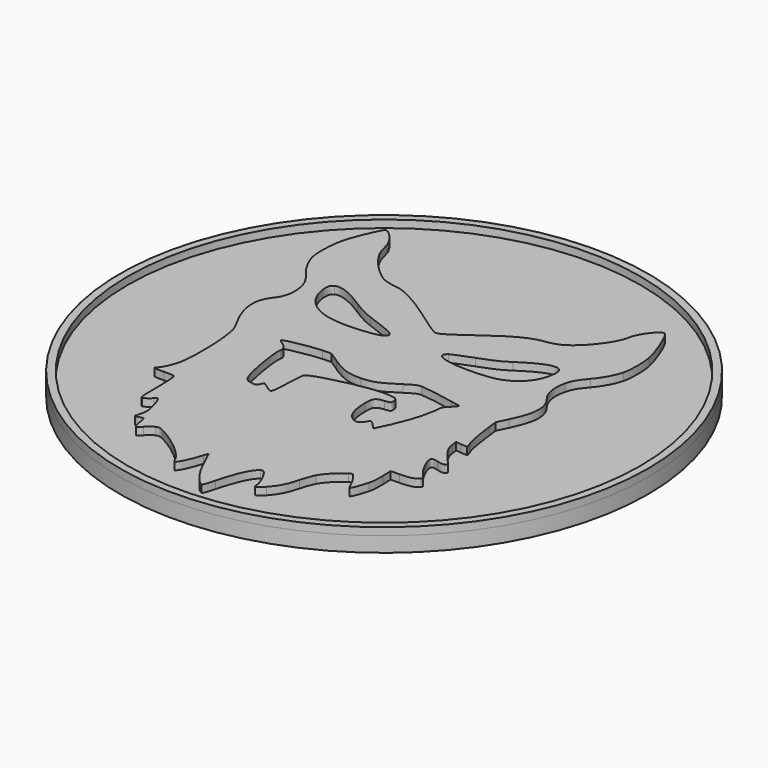
from build123d import *

# Parameters (mm, degrees)
F1_DEPTH = 1
F2_R     = 35
F3_DEPTH = 2
F4_R     = 35
F4_R_2   = 34
F5_DEPTH = 1


# Not quite as in the source:
# - ends of sketch curves that miss each other by under 0.0002 mm in the source are joined


with BuildPart() as f1:
    # F0 (on Top) → F1 (new body)
    with BuildSketch(Plane.XY):
        with BuildLine():
            Line((16.1826469271, 5.2708612479), (16.8400695237, 6.6341461731))
            add(Edge.make_bspline(
                [(16.9910679139, 12.732516303), (18.2577822603, 11.1594923939), (18.2164007999, 9.4882145174), (16.8400695237, 6.6341461731)],
                knots=[0, 0, 0, 0, 1, 1, 1, 1], degree=3))
            add(Edge.make_bspline(
                [(16.3616295009, 16.5726861761), (15.9908697191, 15.1813152196), (16.2392131876, 13.6661808871), (16.9910679139, 12.732516303)],
                knots=[0, 0, 0, 0, 1, 1, 1, 1], degree=3))
            add(Edge.make_bspline(
                [(17.7549925553, 18.9896539173), (16.8340840828, 17.8901305075), (16.608350267, 17.4985672419), (16.3616295009, 16.5726861761)],
                knots=[0, 0, 0, 0, 1, 1, 1, 1], degree=3))
            add(Edge.make_bspline(
                [(19.5483031014, 22.2723542054), (19.2596321814, 21.164071897), (18.6659092272, 20.0772477822), (17.7549925553, 18.9896539173)],
                knots=[0, 0, 0, 0, 1, 1, 1, 1], degree=3))
            add(Edge.make_bspline(
                [(19.5540287341, 26.4991346279), (19.8011714908, 25.3242562633), (19.7983403369, 23.2322956616), (19.5483031014, 22.2723542054)],
                knots=[0, 0, 0, 0, 1, 1, 1, 1], degree=3))
            add(Edge.make_bspline(
                [(17.3613460741, 31.7822766885), (17.7671351183, 31.7076772357), (19.1688004281, 28.330447016), (19.5540287341, 26.4991346279)],
                knots=[0, 0, 0, 0, 1, 1, 1, 1], degree=3))
            add(Edge.make_bspline(
                [(15.074723812, 28.6660865937), (15.2559545981, 29.8714277868), (16.741702099, 31.8961907452), (17.3613460741, 31.7822766885)],
                knots=[0, 0, 0, 0, 1, 1, 1, 1], degree=3))
            add(Edge.make_bspline(
                [(10.5930521191, 23.0509721747), (12.3876829908, 23.8999686358), (14.8154555549, 26.9417409854), (15.074723812, 28.6660865937)],
                knots=[0, 0, 0, 0, 1, 1, 1, 1], degree=3))
            add(Edge.make_bspline(
                [(8.8818992128, 22.5780426556), (9.427403017, 22.6472056597), (10.1781785803, 22.85470593), (10.5930521191, 23.0509721747)],
                knots=[0, 0, 0, 0, 1, 1, 1, 1], degree=3))
            add(Edge.make_bspline(
                [(1.7025667495, 18.7230730334), (5.4136975729, 21.4603613385), (7.0665795458, 22.3478826003), (8.8818992128, 22.5780426556)],
                knots=[0, 0, 0, 0, 1, 1, 1, 1], degree=3))
            add(Edge.make_bspline(
                [(-1.139369586, 17.0344307466), (-0.7369789819, 17.0344307466), (0.035244045, 17.4932769684), (1.7025667495, 18.7230730334)],
                knots=[0, 0, 0, 0, 1, 1, 1, 1], degree=3))
            add(Edge.make_bspline(
                [(-5.4533025812, 19.8115778984), (-2.3041017073, 17.5624688206), (-1.4838653366, 17.0344307466), (-1.139369586, 17.0344307466)],
                knots=[0, 0, 0, 0, 1, 1, 1, 1], degree=3))
            add(Edge.make_bspline(
                [(-8.5535875545, 21.720697149), (-7.7554292585, 21.3184456839), (-6.3603008446, 20.459341854), (-5.4533025812, 19.8115778984)],
                knots=[0, 0, 0, 0, 1, 1, 1, 1], degree=3))
            add(Edge.make_bspline(
                [(-11.0602009371, 22.5804912211), (-10.1866699201, 22.4741962137), (-9.7546933625, 22.3260237003), (-8.5535875545, 21.720697149)],
                knots=[0, 0, 0, 0, 1, 1, 1, 1], degree=3))
            add(Edge.make_bspline(
                [(-12.8320138873, 23.059260006), (-12.3873644201, 22.8418119108), (-11.7152713629, 22.6602027579), (-11.0602009371, 22.5804912211)],
                knots=[0, 0, 0, 0, 1, 1, 1, 1], degree=3))
            add(Edge.make_bspline(
                [(-16.2851561458, 26.3947741984), (-15.4734223835, 25.1582984045), (-13.7806207016, 23.5231600881), (-12.8320138873, 23.059260006)],
                knots=[0, 0, 0, 0, 1, 1, 1, 1], degree=3))
            add(Edge.make_bspline(
                [(-17.4473262444, 29.2439608911), (-17.0559172454, 27.7278100169), (-16.8846759732, 27.3079939642), (-16.2851561458, 26.3947741984)],
                knots=[0, 0, 0, 0, 1, 1, 1, 1], degree=3))
            add(Edge.make_bspline(
                [(-19.6386539259, 31.8102562987), (-19.0337263219, 31.8102562987), (-17.709473149, 30.2594038688), (-17.4473262444, 29.2439608911)],
                knots=[0, 0, 0, 0, 1, 1, 1, 1], degree=3))
            add(Edge.make_bspline(
                [(-21.5027325882, 27.6163899087), (-21.0601702065, 29.0864711639), (-19.8495088364, 31.8102562987), (-19.6386539259, 31.8102562987)],
                knots=[0, 0, 0, 0, 1, 1, 1, 1], degree=3))
            add(Edge.make_bspline(
                [(-21.74919724, 22.2310686119), (-22.0889620877, 23.4073232392), (-21.9668940617, 26.0745641014), (-21.5027325882, 27.6163899087)],
                knots=[0, 0, 0, 0, 1, 1, 1, 1], degree=3))
            add(Edge.make_bspline(
                [(-19.8346130445, 18.8263532445), (-20.7277127085, 19.8575266723), (-21.4183494276, 21.0856880736), (-21.74919724, 22.2310686119)],
                knots=[0, 0, 0, 0, 1, 1, 1, 1], degree=3))
            add(Edge.make_bspline(
                [(-18.7756283455, 17.195879164), (-18.9366280351, 17.6261934412), (-19.3608485153, 18.2793468794), (-19.8346130445, 18.8263532445)],
                knots=[0, 0, 0, 0, 1, 1, 1, 1], degree=3))
            add(Edge.make_bspline(
                [(-19.1345514591, 12.8525804454), (-18.3164443905, 13.9243594269), (-18.1780726475, 15.5987718895), (-18.7756283455, 17.195879164)],
                knots=[0, 0, 0, 0, 1, 1, 1, 1], degree=3))
            add(Edge.make_bspline(
                [(-20.0927388136, 10.3061527194), (-20.0912216529, 11.2790590836), (-19.8535934729, 11.9105845821), (-19.1345514591, 12.8525804454)],
                knots=[0, 0, 0, 0, 1, 1, 1, 1], degree=3))
            add(Edge.make_bspline(
                [(-18.5868828204, 5.7128167654), (-19.6253029115, 7.5160176163), (-20.0948470074, 8.9482768021), (-20.0927388136, 10.3061527194)],
                knots=[0, 0, 0, 0, 1, 1, 1, 1], degree=3))
            add(Edge.make_bspline(
                [(-17.7742137836, 3.1161301218), (-17.9802957504, 4.5409222382), (-18.0615731731, 4.8006232159), (-18.5868828204, 5.7128167654)],
                knots=[0, 0, 0, 0, 1, 1, 1, 1], degree=3))
            add(Edge.make_bspline(
                [(-17.7515684226, -4.5522716364), (-17.4512789538, -3.2317680053), (-17.4636851949, 0.9692171667), (-17.7742137836, 3.1161301218)],
                knots=[0, 0, 0, 0, 1, 1, 1, 1], degree=3))
            add(Edge.make_bspline(
                [(-18.8336035865, -6.9677459637), (-18.4850643607, -6.6784840106), (-17.9773312623, -5.5450502556), (-17.7515684226, -4.5522716364)],
                knots=[0, 0, 0, 0, 1, 1, 1, 1], degree=3))
            add(Edge.make_bspline(
                [(-17.7018741526, -7.3570784314), (-19.0362171041, -7.3929124486), (-19.2551487627, -7.3175965441), (-18.8336035865, -6.9677459637)],
                knots=[0, 0, 0, 0, 1, 1, 1, 1], degree=3))
            add(Edge.make_bspline(
                [(-16.2312680038, -7.6434167057), (-16.3592688758, -7.3277364549), (-16.3895737437, -7.3218366785), (-17.7018741526, -7.3570784314)],
                knots=[0, 0, 0, 0, 1, 1, 1, 1], degree=3))
            add(Edge.make_bspline(
                [(-16.0870003543, -10.6370017437), (-16.0944674236, -9.167807038), (-16.1593848404, -7.8206949583), (-16.2312680038, -7.6434167057)],
                knots=[0, 0, 0, 0, 1, 1, 1, 1], degree=3))
            add(Edge.make_bspline(
                [(-15.8719105864, -13.3085239015), (-16.0455582074, -13.3082600475), (-16.0753051119, -12.9388288587), (-16.0870003543, -10.6370017437)],
                knots=[0, 0, 0, 0, 1, 1, 1, 1], degree=3))
            add(Edge.make_bspline(
                [(-14.808504925, -12.599234109), (-15.0990701411, -12.9541719712), (-15.6308007644, -13.3088352493), (-15.8719105864, -13.3085239015)],
                knots=[0, 0, 0, 0, 1, 1, 1, 1], degree=3))
            add(Edge.make_bspline(
                [(-14.4542465749, -12.4327752793), (-14.5338604857, -12.3835703706), (-14.693277227, -12.4584773013), (-14.808504925, -12.599234109)],
                knots=[0, 0, 0, 0, 1, 1, 1, 1], degree=3))
            add(Edge.make_bspline(
                [(-13.6465008785, -14.7381748021), (-13.7897486442, -13.8486925771), (-14.2393005195, -12.5656191042), (-14.4542465749, -12.4327752793)],
                knots=[0, 0, 0, 0, 1, 1, 1, 1], degree=3))
            add(Edge.make_bspline(
                [(-13.8425972012, -16.7267398007), (-13.5642009335, -15.802671588), (-13.5303510987, -15.4594025828), (-13.6465008785, -14.7381748021)],
                knots=[0, 0, 0, 0, 1, 1, 1, 1], degree=3))
            add(Edge.make_bspline(
                [(-13.6206313971, -16.9565804166), (-13.9077388939, -17.0359609046), (-13.9290952399, -17.0138472975), (-13.8425972012, -16.7267398007)],
                knots=[0, 0, 0, 0, 1, 1, 1, 1], degree=3))
            add(Edge.make_bspline(
                [(-12.6213355831, -17.6683346059), (-12.7824700142, -16.6450057346), (-12.701721355, -16.702519407), (-13.6206313971, -16.9565804166)],
                knots=[0, 0, 0, 0, 1, 1, 1, 1], degree=3))
            add(Edge.make_bspline(
                [(-11.6474622818, -18.296259728), (-12.2924204136, -19.0507966186), (-12.4162194979, -18.9709740871), (-12.6213355831, -17.6683346059)],
                knots=[0, 0, 0, 0, 1, 1, 1, 1], degree=3))
            add(Edge.make_bspline(
                [(-10.658088787, -17.5283588062), (-10.9263820835, -17.6169041763), (-11.3434878275, -17.9406398911), (-11.6474622818, -18.296259728)],
                knots=[0, 0, 0, 0, 1, 1, 1, 1], degree=3))
            add(Edge.make_bspline(
                [(-9.5058434701, -17.7337586224), (-10.1211299837, -17.4133501071), (-10.2435093575, -17.3915358864), (-10.658088787, -17.5283588062)],
                knots=[0, 0, 0, 0, 1, 1, 1, 1], degree=3))
            add(Edge.make_bspline(
                [(-4.6086570732, -21.8510584398), (-5.0797459466, -20.7980697358), (-7.4529784733, -18.8027790978), (-9.5058434701, -17.7337586224)],
                knots=[0, 0, 0, 0, 1, 1, 1, 1], degree=3))
            add(Edge.make_bspline(
                [(-4.2485912957, -22.4117482754), (-4.3086641763, -22.4117482754), (-4.4706930726, -22.1594378494), (-4.6086570732, -21.8510584398)],
                knots=[0, 0, 0, 0, 1, 1, 1, 1], degree=3))
            add(Edge.make_bspline(
                [(-2.8097964453, -19.3936274502), (-3.1152643135, -20.6004416524), (-3.9787477687, -22.4117482754), (-4.2485912957, -22.4117482754)],
                knots=[0, 0, 0, 0, 1, 1, 1, 1], degree=3))
            add(Edge.make_bspline(
                [(-2.5509412078, -18.9318828797), (-2.6140827109, -18.8670367036), (-2.7278935127, -19.0700526865), (-2.8097964453, -19.3936274502)],
                knots=[0, 0, 0, 0, 1, 1, 1, 1], degree=3))
            add(Edge.make_bspline(
                [(-1.8968007795, -20.3001599234), (-2.1945996421, -19.6112567253), (-2.488963125, -18.995532214), (-2.5509412078, -18.9318828797)],
                knots=[0, 0, 0, 0, 1, 1, 1, 1], degree=3))
            add(Edge.make_bspline(
                [(0.3338371083, -24.0328754145), (-0.4071362774, -23.2407141691), (-1.197066549, -21.9188569668), (-1.8968007795, -20.3001599234)],
                knots=[0, 0, 0, 0, 1, 1, 1, 1], degree=3))
            add(Edge.make_bspline(
                [(1.1204531972, -24.6267765581), (1.0130223861, -24.6478043179), (0.6590449526, -24.3805491991), (0.3338371083, -24.0328754145)],
                knots=[0, 0, 0, 0, 1, 1, 1, 1], degree=3))
            add(Edge.make_bspline(
                [(1.6939241225, -23.0929414825), (1.4421320817, -24.0888163409), (1.2505174078, -24.6013185131), (1.1204531972, -24.6267765581)],
                knots=[0, 0, 0, 0, 1, 1, 1, 1], degree=3))
            add(Edge.make_bspline(
                [(3.9030605445, -18.327605588), (3.1741702666, -18.7176953168), (2.3514193669, -20.4924555166), (1.6939241225, -23.0929414825)],
                knots=[0, 0, 0, 0, 1, 1, 1, 1], degree=3))
            add(Edge.make_bspline(
                [(4.4420774092, -18.4852465916), (4.2178581157, -18.2445759986), (4.1146199453, -18.2143831808), (3.9030605445, -18.327605588)],
                knots=[0, 0, 0, 0, 1, 1, 1, 1], degree=3))
            add(Edge.make_bspline(
                [(5.6285669347, -21.0364539456), (5.6285669347, -20.5598781395), (4.8846462994, -18.9602894057), (4.4420774092, -18.4852465916)],
                knots=[0, 0, 0, 0, 1, 1, 1, 1], degree=3))
            add(Edge.make_bspline(
                [(6.6816652261, -20.8641875126), (5.8866518944, -21.7285733485), (5.6285669347, -21.7707912263), (5.6285669347, -21.0364539456)],
                knots=[0, 0, 0, 0, 1, 1, 1, 1], degree=3))
            add(Edge.make_bspline(
                [(8.4073656369, -17.5304485302), (8.0457220123, -18.9941193635), (7.5875116787, -19.8792983051), (6.6816652261, -20.8641875126)],
                knots=[0, 0, 0, 0, 1, 1, 1, 1], degree=3))
            add(Edge.make_bspline(
                [(9.0907778565, -15.6449475583), (8.8672896146, -16.0652142737), (8.5597545379, -16.913689711), (8.4073656369, -17.5304485302)],
                knots=[0, 0, 0, 0, 1, 1, 1, 1], degree=3))
            add(Edge.make_bspline(
                [(11.4702056762, -13.2237648368), (10.7434501534, -13.5995839319), (9.5122292765, -14.8524104089), (9.0907778565, -15.6449475583)],
                knots=[0, 0, 0, 0, 1, 1, 1, 1], degree=3))
            Line((11.4702056762, -13.2237648368), (11.8853471147, -13.0090865054))
            Line((11.8853471147, -13.0090865054), (12.3092523773, -13.4994724319))
            add(Edge.make_bspline(
                [(13.1020663976, -14.8366635997), (12.8991666864, -14.3709204092), (12.5424004916, -13.7691840319), (12.3092523773, -13.4994724319)],
                knots=[0, 0, 0, 0, 1, 1, 1, 1], degree=3))
            add(Edge.make_bspline(
                [(13.5559560333, -15.6834702482), (13.5092169286, -15.6834702482), (13.3049662847, -15.3024067903), (13.1020663976, -14.8366635997)],
                knots=[0, 0, 0, 0, 1, 1, 1, 1], degree=3))
            add(Edge.make_bspline(
                [(14.4159935547, -13.5175121327), (14.1791370598, -14.4315883687), (13.6820492406, -15.6834702482), (13.5559560333, -15.6834702482)],
                knots=[0, 0, 0, 0, 1, 1, 1, 1], degree=3))
            add(Edge.make_bspline(
                [(14.5783865696, -11.3987312954), (14.6090054237, -12.3014524849), (14.5577201139, -12.9705690926), (14.4159935547, -13.5175121327)],
                knots=[0, 0, 0, 0, 1, 1, 1, 1], degree=3))
            Line((14.5783865696, -11.3987312954), (14.5336369243, -10.0793449982))
            Line((14.5336369243, -10.0793449982), (15.7209801056, -10.0660084078))
            add(Edge.make_bspline(
                [(18.0177542399, -9.4314895732), (17.6680936344, -9.8531059899), (16.9473036756, -10.0522352269), (15.7209801056, -10.0660084078)],
                knots=[0, 0, 0, 0, 1, 1, 1, 1], degree=3))
            add(Edge.make_bspline(
                [(17.7291797146, -8.7184359907), (18.1499820536, -9.1519467717), (18.182648591, -9.2326623611), (18.0177542399, -9.4314895732)],
                knots=[0, 0, 0, 0, 1, 1, 1, 1], degree=3))
            add(Edge.make_bspline(
                [(16.1476347273, -5.2435507521), (15.7985795788, -5.5926059006), (16.7728539383, -7.7332287512), (17.7291797146, -8.7184359907)],
                knots=[0, 0, 0, 0, 1, 1, 1, 1], degree=3))
            add(Edge.make_bspline(
                [(16.9577378715, -5.3467150433), (16.5693063774, -5.2328502395), (16.2047603583, -5.1864251211), (16.1476347273, -5.2435507521)],
                knots=[0, 0, 0, 0, 1, 1, 1, 1], degree=3))
            add(Edge.make_bspline(
                [(17.9857316822, -5.4071428956), (17.737751101, -5.5201304728), (17.5020476483, -5.5062754971), (16.9577378715, -5.3467150433)],
                knots=[0, 0, 0, 0, 1, 1, 1, 1], degree=3))
            add(Edge.make_bspline(
                [(17.3823857953, -4.2107087114), (18.3065266557, -5.2594544665), (18.3071519898, -5.2606933491), (17.9857316822, -5.4071428956)],
                knots=[0, 0, 0, 0, 1, 1, 1, 1], degree=3))
            add(Edge.make_bspline(
                [(15.8248052632, -1.40571458), (15.9336608861, -2.324829021), (16.2967345997, -2.9786778026), (17.3823857953, -4.2107087114)],
                knots=[0, 0, 0, 0, 1, 1, 1, 1], degree=3))
            Line((15.8248052632, -1.40571458), (15.7453086794, -0.7344924171))
            Line((15.7453086794, -0.7344924171), (16.4710181089, -0.819784467))
            add(Edge.make_bspline(
                [(17.2721700928, -0.8296394154), (17.2306764064, -0.8711318704), (16.8701580313, -0.8667003539), (16.4710181089, -0.819784467)],
                knots=[0, 0, 0, 0, 1, 1, 1, 1], degree=3))
            add(Edge.make_bspline(
                [(17.1665282121, -0.3208009444), (17.2661251967, -0.559169323), (17.3136637792, -0.788145729), (17.2721700928, -0.8296394154)],
                knots=[0, 0, 0, 0, 1, 1, 1, 1], degree=3))
            add(Edge.make_bspline(
                [(16.3172559356, 4.0615692804), (16.5438485083, 2.0259248054), (16.853390107, 0.4286435632), (17.1665282121, -0.3208009444)],
                knots=[0, 0, 0, 0, 1, 1, 1, 1], degree=3))
            Line((16.3172559356, 4.0615692804), (16.1826469271, 5.2708612479))
        make_face()
        with BuildLine():
            Line((-6.7066094484, 6.6781596656), (-5.3408916131, 5.769749783))
            add(Edge.make_bspline(
                [(-0.8410403768, 4.2604031767), (-2.4856440171, 4.1933010485), (-3.4644012567, 4.5215975683), (-5.3408916131, 5.769749783)],
                knots=[0, 0, 0, 0, 1, 1, 1, 1], degree=3))
            add(Edge.make_bspline(
                [(3.3672639304, 5.9316400679), (1.3503636465, 4.6045031463), (0.6356029284, 4.3206516083), (-0.8410403768, 4.2604031767)],
                knots=[0, 0, 0, 0, 1, 1, 1, 1], degree=3))
            add(Edge.make_bspline(
                [(5.2142422123, 6.7432485874), (4.6851239199, 6.7440401496), (4.4344309191, 6.6338441482), (3.3672639304, 5.9316400679)],
                knots=[0, 0, 0, 0, 1, 1, 1, 1], degree=3))
            add(Edge.make_bspline(
                [(9.7183045591, 6.0295128543), (7.8757827718, 6.4180760995), (5.8293150042, 6.7423699535), (5.2142422123, 6.7432485874)],
                knots=[0, 0, 0, 0, 1, 1, 1, 1], degree=3))
            add(Edge.make_bspline(
                [(10.8067024752, 5.8207422148), (10.7522825794, 5.8208016699), (10.2625035172, 5.9147481323), (9.7183045591, 6.0295128543)],
                knots=[0, 0, 0, 0, 1, 1, 1, 1], degree=3))
            add(Edge.make_bspline(
                [(10.3119761497, 4.9835030897), (10.8625591442, 5.5110540892), (11.0454006713, 5.8204809993), (10.8067024752, 5.8207422148)],
                knots=[0, 0, 0, 0, 1, 1, 1, 1], degree=3))
            add(Edge.make_bspline(
                [(9.7154496584, 3.8973254174), (9.7178771155, 4.3364986819), (9.8080057858, 4.5006144878), (10.3119761497, 4.9835030897)],
                knots=[0, 0, 0, 0, 1, 1, 1, 1], degree=3))
            add(Edge.make_bspline(
                [(8.9394127092, 0.3694162468), (9.3041606647, 1.4118217652), (9.7119641465, 3.2657195314), (9.7154496584, 3.8973254174)],
                knots=[0, 0, 0, 0, 1, 1, 1, 1], degree=3))
            add(Edge.make_bspline(
                [(7.1783664111, -3.677801299), (7.2854990671, -3.6774055179), (8.5001089249, -0.8860633706), (8.9394127092, 0.3694162468)],
                knots=[0, 0, 0, 0, 1, 1, 1, 1], degree=3))
            add(Edge.make_bspline(
                [(6.6023255475, -3.1504033349), (6.8645384156, -3.4406427792), (7.1237579476, -3.6779715728), (7.1783664111, -3.677801299)],
                knots=[0, 0, 0, 0, 1, 1, 1, 1], degree=3))
            add(Edge.make_bspline(
                [(5.976015212, -2.6235290331), (6.0582717091, -2.623133252), (6.340111448, -2.8601638906), (6.6023255475, -3.1504033349)],
                knots=[0, 0, 0, 0, 1, 1, 1, 1], degree=3))
            add(Edge.make_bspline(
                [(5.6016960393, -3.0193549487), (5.7253144716, -2.8021093174), (5.893758715, -2.6239881391), (5.976015212, -2.6235290331)],
                knots=[0, 0, 0, 0, 1, 1, 1, 1], degree=3))
            add(Edge.make_bspline(
                [(4.2854510124, -3.4573236316), (4.8201644177, -3.7696145894), (5.2576001155, -3.6240609153), (5.6016960393, -3.0193549487)],
                knots=[0, 0, 0, 0, 1, 1, 1, 1], degree=3))
            add(Edge.make_bspline(
                [(2.9339522713, 0.1769491484), (2.9528391194, -1.768404474), (3.3854343268, -2.9316868053), (4.2854510124, -3.4573236316)],
                knots=[0, 0, 0, 0, 1, 1, 1, 1], degree=3))
            add(Edge.make_bspline(
                [(4.2212711556, 1.8225724966), (3.1161172766, 1.7085098022), (2.9214983606, 1.4597218276), (2.9339522713, 0.1769491484)],
                knots=[0, 0, 0, 0, 1, 1, 1, 1], degree=3))
            add(Edge.make_bspline(
                [(4.9689320099, 2.3268714467), (4.9689320099, 1.9046337417), (4.9603565777, 1.8988526996), (4.2212711556, 1.8225724966)],
                knots=[0, 0, 0, 0, 1, 1, 1, 1], degree=3))
            add(Edge.make_bspline(
                [(3.6235124659, 3.1423348737), (4.7379647372, 3.0580493391), (4.9689320099, 2.9180589395), (4.9689320099, 2.3268714467)],
                knots=[0, 0, 0, 0, 1, 1, 1, 1], degree=3))
            add(Edge.make_bspline(
                [(-3.8675741001, 1.9066351625), (-0.8988150888, 2.7667017078), (2.0841338169, 3.2587578305), (3.6235124659, 3.1423348737)],
                knots=[0, 0, 0, 0, 1, 1, 1, 1], degree=3))
            add(Edge.make_bspline(
                [(-5.9239390328, 0.9621260015), (-5.7990002749, 1.251551544), (-5.2356982843, 1.5102801316), (-3.8675741001, 1.9066351625)],
                knots=[0, 0, 0, 0, 1, 1, 1, 1], degree=3))
            add(Edge.make_bspline(
                [(-6.0990524509, -1.4998327234), (-6.0551351773, -0.2671303941), (-5.9763339368, 0.8407505044), (-5.9239390328, 0.9621260015)],
                knots=[0, 0, 0, 0, 1, 1, 1, 1], degree=3))
            add(Edge.make_bspline(
                [(-7.2172699194, -3.3544640039), (-6.2140942197, -4.1202053683), (-6.1910451621, -4.0819769637), (-6.0990524509, -1.4998327234)],
                knots=[0, 0, 0, 0, 1, 1, 1, 1], degree=3))
            add(Edge.make_bspline(
                [(-7.9481521194, -2.8865492946), (-7.8833179046, -2.8865492946), (-7.5544212049, -3.0971113272), (-7.2172699194, -3.3544640039)],
                knots=[0, 0, 0, 0, 1, 1, 1, 1], degree=3))
            add(Edge.make_bspline(
                [(-8.2040022353, -3.282330355), (-8.1281178133, -3.0646507718), (-8.0129851029, -2.8865492946), (-7.9481521194, -2.8865492946)],
                knots=[0, 0, 0, 0, 1, 1, 1, 1], degree=3))
            add(Edge.make_bspline(
                [(-9.4286860404, -3.543502231), (-8.6034177972, -3.7727333442), (-8.3566087279, -3.7200997402), (-8.2040022353, -3.282330355)],
                knots=[0, 0, 0, 0, 1, 1, 1, 1], degree=3))
            add(Edge.make_bspline(
                [(-10.2002017625, -2.7311325806), (-9.9525984926, -3.3067025527), (-9.8348523958, -3.4306835205), (-9.4286860404, -3.543502231)],
                knots=[0, 0, 0, 0, 1, 1, 1, 1], degree=3))
            add(Edge.make_bspline(
                [(-11.3050629395, 3.9402110218), (-11.5125498411, 3.1467820456), (-10.7512201162, -1.4502557806), (-10.2002017625, -2.7311325806)],
                knots=[0, 0, 0, 0, 1, 1, 1, 1], degree=3))
            add(Edge.make_bspline(
                [(-12.1093440564, 5.2639310336), (-11.508233189, 4.8989167615), (-11.1909249587, 4.376676968), (-11.3050629395, 3.9402110218)],
                knots=[0, 0, 0, 0, 1, 1, 1, 1], degree=3))
            add(Edge.make_bspline(
                [(-12.6625008591, 5.7546705246), (-12.6832582565, 5.6821106635), (-12.4343383549, 5.4612780245), (-12.1093440564, 5.2639310336)],
                knots=[0, 0, 0, 0, 1, 1, 1, 1], degree=3))
            add(Edge.make_bspline(
                [(-7.8939526297, 6.6489629847), (-9.1710167388, 6.6175590768), (-12.5995941861, 5.9745652504), (-12.6625008591, 5.7546705246)],
                knots=[0, 0, 0, 0, 1, 1, 1, 1], degree=3))
            Line((-7.8939526297, 6.6489629847), (-6.7066094484, 6.6781596656))
        make_face(mode=Mode.SUBTRACT)
        with BuildLine():
            add(Edge.make_bspline(
                [(-7.3859715085, 12.6826176341), (-5.599954064, 12.8305896184), (-4.6617404603, 13.146136535), (-4.6617404603, 13.5988493817)],
                knots=[0, 0, 0, 0, 1, 1, 1, 1], degree=3))
            add(Edge.make_bspline(
                [(-11.156274239, 12.6869988425), (-9.8746203009, 12.5376864796), (-9.1454992386, 12.5368395081), (-7.3859715085, 12.6826176341)],
                knots=[0, 0, 0, 0, 1, 1, 1, 1], degree=3))
            add(Edge.make_bspline(
                [(-16.3643044422, 17.3188048915), (-16.0628999263, 14.7739207116), (-14.1022559623, 13.0302043468), (-11.156274239, 12.6869988425)],
                knots=[0, 0, 0, 0, 1, 1, 1, 1], degree=3))
            add(Edge.make_bspline(
                [(-15.9309729061, 18.7302736102), (-16.3439507416, 18.5421087399), (-16.4631876137, 18.1537247395), (-16.3643044422, 17.3188048915)],
                knots=[0, 0, 0, 0, 1, 1, 1, 1], degree=3))
            add(Edge.make_bspline(
                [(-11.4032732831, 16.9712165956), (-13.5242613474, 18.4008518409), (-15.2135460309, 19.0571556964), (-15.9309729061, 18.7302736102)],
                knots=[0, 0, 0, 0, 1, 1, 1, 1], degree=3))
            add(Edge.make_bspline(
                [(-8.6855145746, 15.5825884899), (-9.6868684501, 15.9516886297), (-10.529321331, 16.3821374725), (-11.4032732831, 16.9712165956)],
                knots=[0, 0, 0, 0, 1, 1, 1, 1], degree=3))
            add(Edge.make_bspline(
                [(-4.6617404603, 13.5988493817), (-4.6617404603, 14.048054201), (-5.0746233083, 14.2516084461), (-8.6855145746, 15.5825884899)],
                knots=[0, 0, 0, 0, 1, 1, 1, 1], degree=3))
        make_face(mode=Mode.SUBTRACT)
        with BuildLine():
            add(Edge.make_bspline(
                [(10.0739615115, 12.8910028708), (12.308011032, 13.4728986556), (13.7436077955, 14.9711741222), (14.1105114384, 17.1037888268)],
                knots=[0, 0, 0, 0, 1, 1, 1, 1], degree=3))
            add(Edge.make_bspline(
                [(7.7759840269, 12.6331409558), (8.6305453456, 12.6683484076), (9.6646341846, 12.7843873687), (10.0739615115, 12.8910028708)],
                knots=[0, 0, 0, 0, 1, 1, 1, 1], degree=3))
            add(Edge.make_bspline(
                [(2.8407644772, 14.1196919802), (1.5237871674, 13.1819230585), (3.8787583561, 12.4725752181), (7.7759840269, 12.6331409558)],
                knots=[0, 0, 0, 0, 1, 1, 1, 1], degree=3))
            add(Edge.make_bspline(
                [(5.5532209509, 15.2408051588), (4.2695142283, 14.7724049581), (3.0489083754, 14.2679040717), (2.8407644772, 14.1196919802)],
                knots=[0, 0, 0, 0, 1, 1, 1, 1], degree=3))
            add(Edge.make_bspline(
                [(9.1655686915, 16.9457574952), (8.1231909657, 16.2499492369), (7.4564145674, 15.9352452459), (5.5532209509, 15.2408051588)],
                knots=[0, 0, 0, 0, 1, 1, 1, 1], degree=3))
            add(Edge.make_bspline(
                [(13.7019927362, 18.7387617947), (12.93348882, 19.0570870943), (11.4502927876, 18.4708602334), (9.1655686915, 16.9457574952)],
                knots=[0, 0, 0, 0, 1, 1, 1, 1], degree=3))
            add(Edge.make_bspline(
                [(14.1105114384, 17.1037888268), (14.2848252029, 18.1169763801), (14.1788126953, 18.5412577227), (13.7019927362, 18.7387617947)],
                knots=[0, 0, 0, 0, 1, 1, 1, 1], degree=3))
        make_face(mode=Mode.SUBTRACT)
    extrude(amount=F1_DEPTH)


with BuildPart() as f3:
    # F2 (on Top) → F3 (new body)
    with BuildSketch(Plane.XY):
        with Locations((0, 7)):
            Circle(F2_R)
    extrude(amount=-F3_DEPTH)

    # F4 (on face) → F5 (join)
    with BuildSketch(Plane.XY):
        with Locations((0, 7)):
            Circle(F4_R)
        with Locations((0, 7)):
            Circle(F4_R_2, mode=Mode.SUBTRACT)
    extrude(amount=F5_DEPTH)


solid = Compound([f1.part, f3.part])
